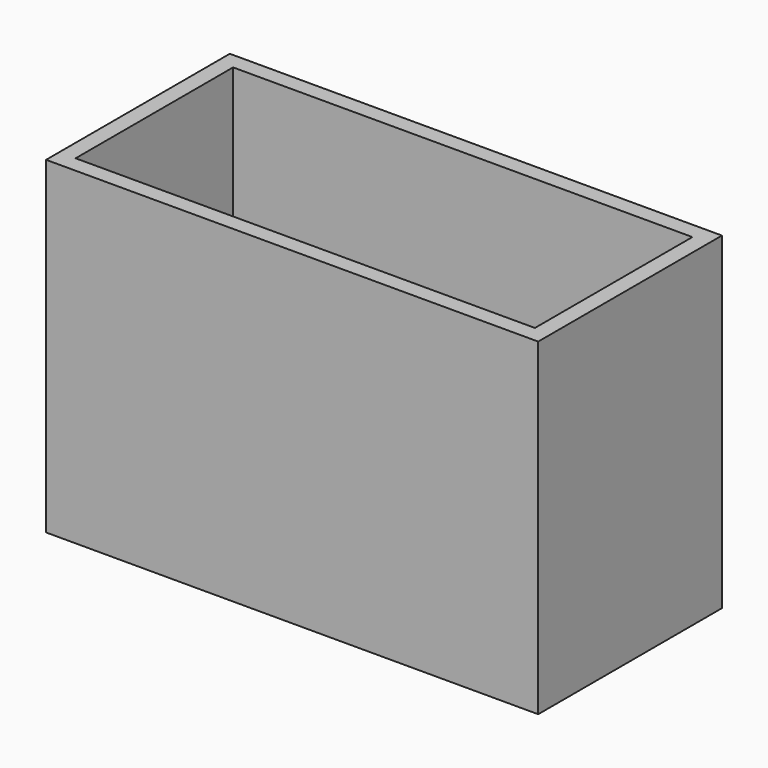
from build123d import *

# Parameters (mm, degrees)
F0_W     = 150
F0_H     = 70
F1_DEPTH = 100
F2_T     = -5


# Not quite as in the source:
# - the program builds the solid bodies; features that only make, move or delete a surface that nothing else refers to are left out


with BuildPart() as f1:
    # F0 (on Top) → F1 (new body)
    with BuildSketch(Plane.XY):
        Rectangle(F0_W, F0_H)
    extrude(amount=F1_DEPTH)

    # F2
    f2_openings = [f1.faces().sort_by_distance(p)[0] for p in [
        (0, 0, 100),
    ]]
    offset(amount=F2_T, openings=f2_openings)


solid = f1.part
